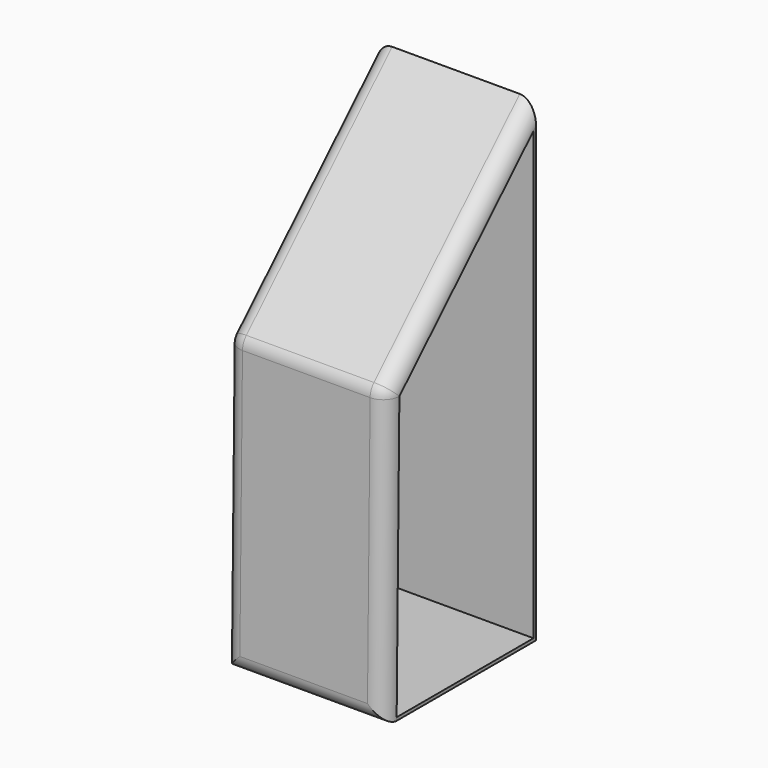
from build123d import *

# Parameters (mm, degrees)
F1_DEPTH = 50
F2_R     = 5.08
F3_T     = -1


# Not quite as in the source:
# - a shell that OpenCascade refuses in one call is made with other operations: the cavity is built on its own and cut out


with BuildPart() as f1:
    # F0 (on Right) → F1 (new body)
    with BuildSketch(Plane.YZ):
        Polygon((40.6505316496, -75.3882825375), (40.6505316496, 73.1709599495), (-17.738416791, 15.5211091042), (-18.8470706344, -75.3882825375), align=None)
    extrude(amount=F1_DEPTH)

    # F2
    f2_edges = [f1.edges().sort_by_distance(p)[0] for p in [
        (50, -18.292744, -29.933587),
        (50, 11.456057, 44.346035),
        (25, -17.738417, 15.521109),
        (0, 11.456057, 44.346035),
        (25, -18.847071, -75.388283),
        (0, -18.292744, -29.933587),
    ]]
    fillet(f2_edges, radius=F2_R)

    # F3: a shell. OpenCascade refuses it in one call, so the cavity is built on its own and cut out:
    # the body offset inwards by the wall thickness, plus a prism from it out through each open face.
    f3_core = offset(f1.part, amount=F3_T, mode=Mode.PRIVATE)
    f3_exits = [f3_core.faces().sort_by_distance(p)[0] for p in [
        (49, 15.243523, -16.834061),
    ]]
    add(f3_core, mode=Mode.SUBTRACT)
    extrude(f3_exits, amount=-F3_T, mode=Mode.SUBTRACT)


solid = f1.part
